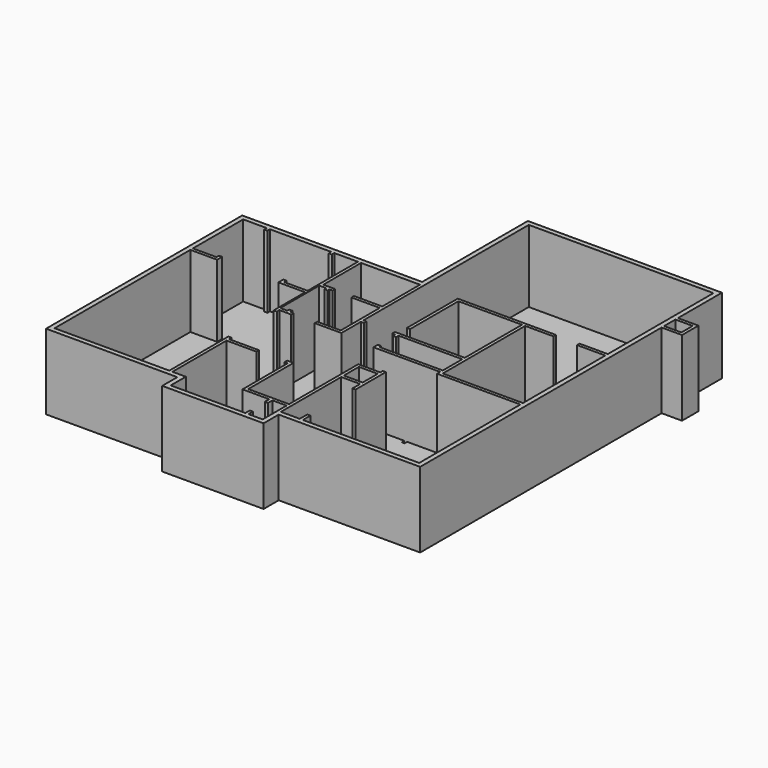
from build123d import *

# Parameters (mm, degrees)
F1_DEPTH = 101.6
F0_W     = 609.6
F0_H     = 609.6
F0_W_2   = 558.8
F0_H_2   = 457.2
F2_DEPTH = 2438.4


with BuildPart() as f1:
    # F0 (on Top) → F1 (new body)
    with BuildSketch(Plane.XY):
        Polygon((5996.5963871956, 9279.5369567871), (27.5963871956, 9279.5369567871), (27.5963871956, 5012.3369567871), (27.5963871956, 2599.3369567871), (129.1963871956, 2599.3369567871), (129.1963871956, 2497.7369567871), (27.5963871956, 2497.7369567871), (27.5963871956, 1710.3369567871), (-836.0036128044, 1710.3369567871), (-836.0036128044, 1811.9369567871), (-74.0036128044, 1811.9369567871), (-74.0036128044, 3386.7369567871), (-988.4036128044, 3386.7369567871), (-988.4036128044, 3488.3369567871), (-74.0036128044, 3488.3369567871), (-74.0036128044, 5012.3369567871), (-1979.0036128044, 5012.3369567871), (-1979.0036128044, 3488.3369567871), (-1598.0036128044, 3488.3369567871), (-1598.0036128044, 3386.7369567871), (-1699.6036128044, 3386.7369567871), (-1699.6036128044, 3310.5369567871), (-1801.2036128044, 3310.5369567871), (-1801.2036128044, 3386.7369567871), (-2029.8036128044, 3386.7369567871), (-2029.8036128044, 1811.9369567871), (-1801.2036128044, 1811.9369567871), (-1801.2036128044, 1888.1369567871), (-1699.6036128044, 1888.1369567871), (-1699.6036128044, 1811.9369567871), (-1598.0036128044, 1811.9369567871), (-1598.0036128044, 1710.3369567871), (-1979.0036128044, 1710.3369567871), (-1979.0036128044, 1608.7369567871), (-2080.6036128044, 1608.7369567871), (-2080.6036128044, 2878.7369567871), (-2944.2036128044, 2878.7369567871), (-2944.2036128044, 3081.9369567871), (-2842.6036128044, 3081.9369567871), (-2842.6036128044, 2980.3369567871), (-2080.6036128044, 2980.3369567871), (-2080.6036128044, 5012.3369567871), (-2842.6036128044, 5012.3369567871), (-2842.6036128044, 4910.7369567871), (-2944.2036128044, 4910.7369567871), (-2944.2036128044, 5012.3369567871), (-4925.4036128044, 5012.3369567871), (-4925.4036128044, 4910.7369567871), (-5027.0036128044, 4910.7369567871), (-5027.0036128044, 5012.3369567871), (-5789.0036128044, 5012.3369567871), (-5789.0036128044, 2980.3369567871), (-5027.0036128044, 2980.3369567871), (-5027.0036128044, 3081.9369567871), (-4925.4036128044, 3081.9369567871), (-4925.4036128044, 2878.7369567871), (-5789.0036128044, 2878.7369567871), (-5789.0036128044, -2607.6630432129), (-2080.6036128044, -2607.6630432129), (-2080.6036128044, -220.0630432129), (-1979.0036128044, -220.0630432129), (-1979.0036128044, -321.6630432129), (-1013.8036128044, -321.6630432129), (-1013.8036128044, -423.2630432129), (-1979.0036128044, -423.2630432129), (-1979.0036128044, -2607.6630432129), (-1547.2036128044, -2607.6630432129), (-1547.2036128044, -3217.2630432129), (865.7963871956, -3217.2630432129), (865.7963871956, -3039.4630432129), (967.3963871956, -3039.4630432129), (967.3963871956, -3217.2630432129), (1424.5963871956, -3217.2630432129), (1424.5963871956, -2607.6630432129), (1424.5963871956, -2252.0630432129), (967.3963871956, -2252.0630432129), (967.3963871956, -2429.8630432129), (865.7963871956, -2429.8630432129), (865.7963871956, -2252.0630432129), (2.1963871956, -2252.0630432129), (2.1963871956, -423.2630432129), (-99.4036128044, -423.2630432129), (-99.4036128044, -321.6630432129), (103.7963871956, -321.6630432129), (103.7963871956, -2150.4630432129), (1424.5963871956, -2150.4630432129), (1424.5963871956, 643.5369567871), (2135.7963871956, 643.5369567871), (2135.7963871956, 745.1369567871), (2237.3963871956, 745.1369567871), (2237.3963871956, -474.0630432129), (2135.7963871956, -474.0630432129), (2135.7963871956, -169.2630432129), (1526.1963871956, -169.2630432129), (1526.1963871956, -2607.6630432129), (2135.7963871956, -2607.6630432129), (2135.7963871956, -2302.8630432129), (2237.3963871956, -2302.8630432129), (2237.3963871956, -2607.6630432129), (5996.5963871956, -2607.6630432129), (5996.5963871956, 1481.7369567871), (3304.1963871956, 1481.7369567871), (3304.1963871956, 1608.7369567871), (2237.3963871956, 1608.7369567871), (2237.3963871956, 1507.1369567871), (2135.7963871956, 1507.1369567871), (2135.7963871956, 1608.7369567871), (1145.1963871956, 1608.7369567871), (1145.1963871956, 1786.5369567871), (1246.7963871956, 1786.5369567871), (1246.7963871956, 1710.3369567871), (3304.1963871956, 1710.3369567871), (3304.1963871956, 2497.7369567871), (1246.7963871956, 2497.7369567871), (1246.7963871956, 2396.1369567871), (1145.1963871956, 2396.1369567871), (1145.1963871956, 2497.7369567871), (1043.5963871956, 2497.7369567871), (1043.5963871956, 2599.3369567871), (1145.1963871956, 2599.3369567871), (1145.1963871956, 2600.1431941986), (1246.7963871956, 2600.1431941986), (1246.7963871956, 2599.3369567871), (3304.1963871956, 2599.3369567871), (3304.1963871956, 4910.7369567871), (1246.7963871956, 4910.7369567871), (1246.7963871956, 2959.5220088959), (1145.1963871956, 2959.5220088959), (1145.1963871956, 5012.3369567871), (4320.1963871956, 5012.3369567871), (4320.1963871956, 4910.7369567871), (3405.7963871956, 4910.7369567871), (3405.7963871956, 2497.7369567871), (3405.7963871956, 1583.3369567871), (5996.5963871956, 1583.3369567871), (5996.5963871956, 4910.7369567871), (5082.1963871956, 4910.7369567871), (5082.1963871956, 5012.3369567871), (5996.5963871956, 5012.3369567871), align=None)
    extrude(amount=F1_DEPTH)

    # F0 (on Top) → F2 (join)
    with BuildSketch(Plane.XY):
        Polygon((6148.9963871956, 9431.9369567871), (-124.8036128044, 9431.9369567871), (-124.8036128044, 5164.7369567871), (-5941.4036128044, 5164.7369567871), (-5941.4036128044, -2760.0630432129), (-1699.6036128044, -2760.0630432129), (-1699.6036128044, -3369.6630432129), (1576.9963871956, -3369.6630432129), (1576.9963871956, -2760.0630432129), (6148.9963871956, -2760.0630432129), (6148.9963871956, 6993.5369567871), (6809.3963871956, 6993.5369567871), (6809.3963871956, 7653.9369567871), (6148.9963871956, 7653.9369567871), align=None)
        with Locations((1830.9963871956, 237.1369567871)):
            Rectangle(F0_W, F0_H, mode=Mode.SUBTRACT)
        Polygon((27.5963871956, 5012.3369567871), (27.5963871956, 9279.5369567871), (5996.5963871956, 9279.5369567871), (5996.5963871956, 5012.3369567871), (5082.1963871956, 5012.3369567871), (5082.1963871956, 4910.7369567871), (5996.5963871956, 4910.7369567871), (5996.5963871956, 1583.3369567871), (3405.7963871956, 1583.3369567871), (3405.7963871956, 2497.7369567871), (3405.7963871956, 4910.7369567871), (4320.1963871956, 4910.7369567871), (4320.1963871956, 5012.3369567871), (1145.1963871956, 5012.3369567871), (1145.1963871956, 2959.5220088959), (1246.7963871956, 2959.5220088959), (1246.7963871956, 4910.7369567871), (3304.1963871956, 4910.7369567871), (3304.1963871956, 2599.3369567871), (1246.7963871956, 2599.3369567871), (1246.7963871956, 2600.1431941986), (1145.1963871956, 2600.1431941986), (1145.1963871956, 2599.3369567871), (1043.5963871956, 2599.3369567871), (1043.5963871956, 2497.7369567871), (1145.1963871956, 2497.7369567871), (1145.1963871956, 2396.1369567871), (1246.7963871956, 2396.1369567871), (1246.7963871956, 2497.7369567871), (3304.1963871956, 2497.7369567871), (3304.1963871956, 1710.3369567871), (1246.7963871956, 1710.3369567871), (1246.7963871956, 1786.5369567871), (1145.1963871956, 1786.5369567871), (1145.1963871956, 1608.7369567871), (2135.7963871956, 1608.7369567871), (2237.3963871956, 1608.7369567871), (3304.1963871956, 1608.7369567871), (3304.1963871956, 1481.7369567871), (5996.5963871956, 1481.7369567871), (5996.5963871956, -2607.6630432129), (2237.3963871956, -2607.6630432129), (2237.3963871956, -2302.8630432129), (2135.7963871956, -2302.8630432129), (2135.7963871956, -2607.6630432129), (1526.1963871956, -2607.6630432129), (1526.1963871956, -169.2630432129), (2135.7963871956, -169.2630432129), (2135.7963871956, -474.0630432129), (2237.3963871956, -474.0630432129), (2237.3963871956, 745.1369567871), (2135.7963871956, 745.1369567871), (2135.7963871956, 643.5369567871), (1424.5963871956, 643.5369567871), (1424.5963871956, -2150.4630432129), (103.7963871956, -2150.4630432129), (103.7963871956, -321.6630432129), (-99.4036128044, -321.6630432129), (-99.4036128044, -423.2630432129), (2.1963871956, -423.2630432129), (2.1963871956, -2252.0630432129), (865.7963871956, -2252.0630432129), (865.7963871956, -2429.8630432129), (967.3963871956, -2429.8630432129), (967.3963871956, -2252.0630432129), (1424.5963871956, -2252.0630432129), (1424.5963871956, -2607.6630432129), (1424.5963871956, -3217.2630432129), (967.3963871956, -3217.2630432129), (967.3963871956, -3039.4630432129), (865.7963871956, -3039.4630432129), (865.7963871956, -3217.2630432129), (-1547.2036128044, -3217.2630432129), (-1547.2036128044, -2607.6630432129), (-1979.0036128044, -2607.6630432129), (-1979.0036128044, -423.2630432129), (-1013.8036128044, -423.2630432129), (-1013.8036128044, -321.6630432129), (-1979.0036128044, -321.6630432129), (-1979.0036128044, -220.0630432129), (-2080.6036128044, -220.0630432129), (-2080.6036128044, -2607.6630432129), (-5789.0036128044, -2607.6630432129), (-5789.0036128044, 2878.7369567871), (-4925.4036128044, 2878.7369567871), (-4925.4036128044, 3081.9369567871), (-5027.0036128044, 3081.9369567871), (-5027.0036128044, 2980.3369567871), (-5789.0036128044, 2980.3369567871), (-5789.0036128044, 5012.3369567871), (-5027.0036128044, 5012.3369567871), (-5027.0036128044, 4910.7369567871), (-4925.4036128044, 4910.7369567871), (-4925.4036128044, 5012.3369567871), (-2944.2036128044, 5012.3369567871), (-2944.2036128044, 4910.7369567871), (-2842.6036128044, 4910.7369567871), (-2842.6036128044, 5012.3369567871), (-2080.6036128044, 5012.3369567871), (-2080.6036128044, 2980.3369567871), (-2842.6036128044, 2980.3369567871), (-2842.6036128044, 3081.9369567871), (-2944.2036128044, 3081.9369567871), (-2944.2036128044, 2878.7369567871), (-2080.6036128044, 2878.7369567871), (-2080.6036128044, 1608.7369567871), (-1979.0036128044, 1608.7369567871), (-1979.0036128044, 1710.3369567871), (-1598.0036128044, 1710.3369567871), (-1598.0036128044, 1811.9369567871), (-1699.6036128044, 1811.9369567871), (-1699.6036128044, 1888.1369567871), (-1801.2036128044, 1888.1369567871), (-1801.2036128044, 1811.9369567871), (-2029.8036128044, 1811.9369567871), (-2029.8036128044, 3386.7369567871), (-1801.2036128044, 3386.7369567871), (-1801.2036128044, 3310.5369567871), (-1699.6036128044, 3310.5369567871), (-1699.6036128044, 3386.7369567871), (-1598.0036128044, 3386.7369567871), (-1598.0036128044, 3488.3369567871), (-1979.0036128044, 3488.3369567871), (-1979.0036128044, 5012.3369567871), (-74.0036128044, 5012.3369567871), (-74.0036128044, 3488.3369567871), (-988.4036128044, 3488.3369567871), (-988.4036128044, 3386.7369567871), (-74.0036128044, 3386.7369567871), (-74.0036128044, 1811.9369567871), (-836.0036128044, 1811.9369567871), (-836.0036128044, 1710.3369567871), (27.5963871956, 1710.3369567871), (27.5963871956, 2497.7369567871), (129.1963871956, 2497.7369567871), (129.1963871956, 2599.3369567871), (27.5963871956, 2599.3369567871), align=None, mode=Mode.SUBTRACT)
        with Locations((6428.3963871956, 7323.7369567871)):
            Rectangle(F0_W_2, F0_H_2, mode=Mode.SUBTRACT)
    extrude(amount=F2_DEPTH)


with BuildPart() as f1b:
    # F0 (on Top) → F1, piece 2 (new body)
    with BuildSketch(Plane.XY):
        with Locations((1830.9963871956, 237.1369567871)):
            Rectangle(F0_W, F0_H)
    extrude(amount=F1_DEPTH)


with BuildPart() as f1c:
    # F0 (on Top) → F1, piece 3 (new body)
    with BuildSketch(Plane.XY):
        with Locations((6428.3963871956, 7323.7369567871)):
            Rectangle(F0_W_2, F0_H_2)
    extrude(amount=F1_DEPTH)


solid = Compound([f1.part, f1b.part, f1c.part])
